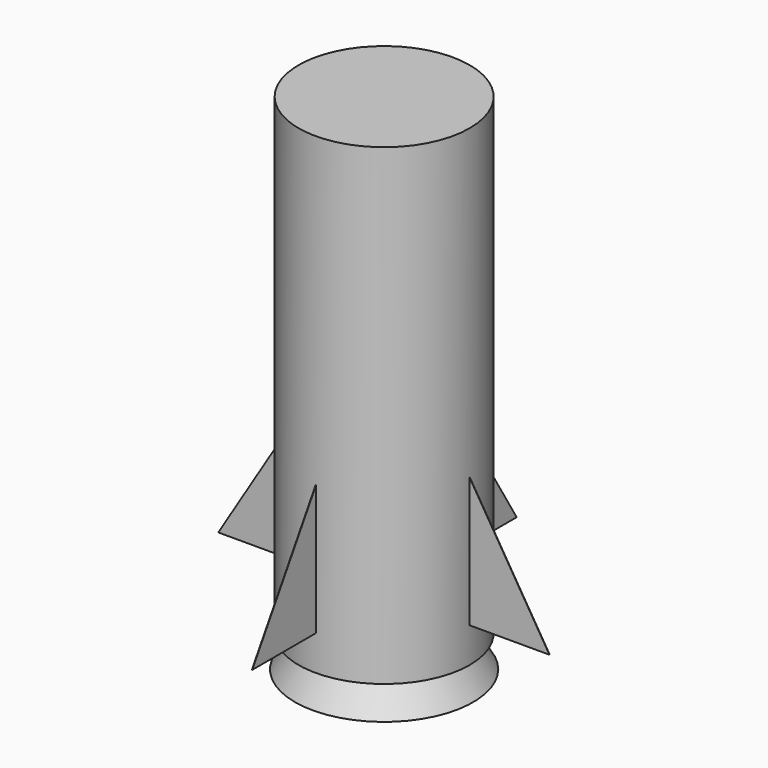
from build123d import *

# Parameters (mm, degrees)
F0_R     = 6.8963363522
F1_DEPTH = 38.1
F3_DEPTH = 2.54
F3_TAPER = -30
F5_DEPTH = 0.0254
F7_DEPTH = 0.0254


# Not quite as in the source:
# - the program builds the solid bodies; features that only make, move or delete a surface that nothing else refers to are left out


with BuildPart() as f1:
    # F0 (on Top) → F1 (new body)
    with BuildSketch(Plane.XY):
        Circle(F0_R)
    extrude(amount=-F1_DEPTH)

    # F2 (on face) → F3 (join)
    with BuildSketch(Plane(origin=(0, 0, -38.1), x_dir=(1, 0, 0), z_dir=(0, 0, -1))):
        with BuildLine():
            Line((-5.7197166772, 0), (5.7197166772, 0))
            ThreePointArc((5.7197166772, 0), (0, 5.7197166772), (-5.7197166772, 0))
        make_face()
        with BuildLine():
            ThreePointArc((-5.7197166772, 0), (0, -5.7197166772), (5.7197166772, 0))
            Line((5.7197166772, 0), (-5.7197166772, 0))
        make_face()
    extrude(amount=F3_DEPTH, taper=F3_TAPER)


with BuildPart() as f5:
    # F4 (on Front) → F5 (new body)
    with BuildSketch(Plane.XZ):
        Polygon((13.350895606, -35.2622419596), (6.9121057168, -24.7766189277), (6.9058611989, -35.2622419596), align=None)
    extrude(amount=F5_DEPTH)


with BuildPart() as f5b:
    # F4 (on Front) → F5, piece 2 (new body)
    with BuildSketch(Plane.XZ):
        Polygon((-13.350895606, -35.2622419596), (-6.9058611989, -35.2622419596), (-6.9121057168, -24.7766189277), align=None)
    extrude(amount=F5_DEPTH)


with BuildPart() as f7:
    # F6 (on Right) → F7 (new body)
    with BuildSketch(Plane.YZ):
        Polygon((6.8963435479, -24.7504599392), (6.8963435479, -35.2618433535), (13.324634172, -35.2618433535), align=None)
    extrude(amount=F7_DEPTH)


with BuildPart() as f7b:
    # F6 (on Right) → F7, piece 2 (new body)
    with BuildSketch(Plane.YZ):
        Polygon((-13.324634172, -35.2618433535), (-6.8963435479, -35.2618433535), (-6.8963435479, -24.7504599392), align=None)
    extrude(amount=F7_DEPTH)


solid = Compound([f1.part, f5.part, f5b.part, f7.part, f7b.part])
